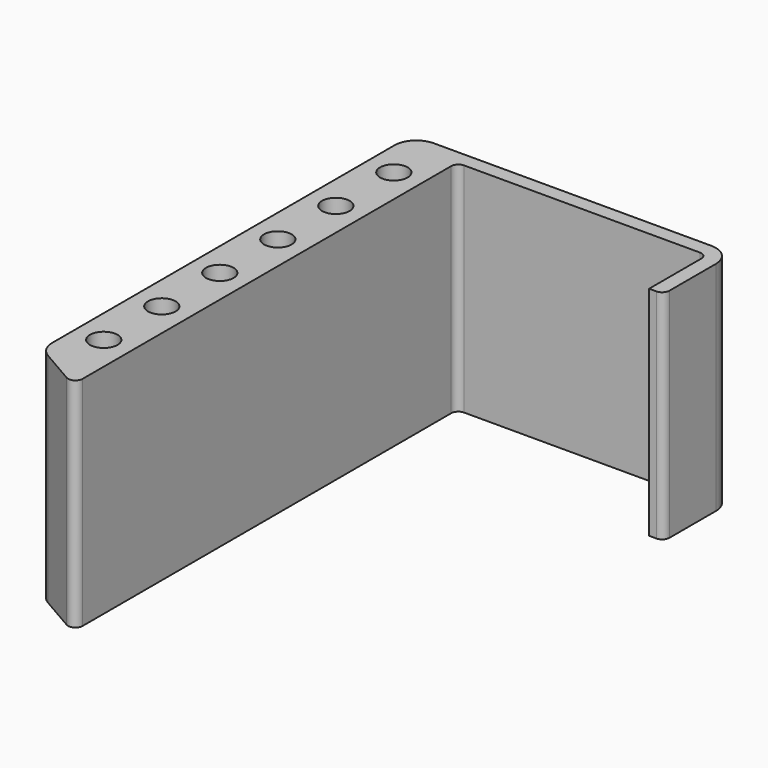
from build123d import *

# Parameters (mm, degrees)
F1_DEPTH  = 15
F2_R      = 1.9
F3_DEPTH  = 15
F4_R      = 1
F5_R      = 3
F7_R      = 1.9
F7_R_2    = 1.5
F8_DEPTH  = 1.6
F9_W      = 2
F9_H      = 58
F10_DEPTH = 12
F11_R     = 0.99999
F12_SIZE  = 0.39999


# Not quite as in the source:
# - a fillet or chamfer is up to 0.001 mm smaller than in the source, because OpenCascade refuses the exact size
# - a feature names something its author has since deleted; it is built from what else it names


with BuildPart() as f1:
    # F0 (on Top) → F1 (new body)
    with BuildSketch(Plane.XY):
        Polygon((-2, 2), (0, 0), (34.5, 0), (34.5, -10), (36.5, -10), (36.5, 2), align=None)
    extrude(amount=F1_DEPTH)

    # F2 (on Top) → F3 (join, through all)
    with BuildSketch(Plane.XY):
        Polygon((0, 0), (-2, 2), (-7.8, 2), (-7.8, -61.7483339502), (0, -66.2516660498), align=None)
        with Locations((-3.9, -56)):
            Circle(F2_R, mode=Mode.SUBTRACT)
        with Locations((-3.9, -46)):
            Circle(F2_R, mode=Mode.SUBTRACT)
        with Locations((-3.9, -36)):
            Circle(F2_R, mode=Mode.SUBTRACT)
        with Locations((-3.9, -26)):
            Circle(F2_R, mode=Mode.SUBTRACT)
        with Locations((-3.9, -16)):
            Circle(F2_R, mode=Mode.SUBTRACT)
        with Locations((-3.9, -6)):
            Circle(F2_R, mode=Mode.SUBTRACT)
    extrude(amount=F3_DEPTH)

    # F4
    f4_edges = [f1.edges().sort_by_distance(p)[0] for p in [
        (34.5, 0, 7.5),
        (0, -66.251666, 7.5),
        (36.5, -10, 7.5),
        (0, 0, 7.5),
    ]]
    fillet(f4_edges, radius=F4_R)

    # F5
    f5_edges = [f1.edges().sort_by_distance(p)[0] for p in [
        (36.5, 2, 7.5),
        (-7.8, 2, 7.5),
        (-7.8, -61.748334, 7.5),
    ]]
    fillet(f5_edges, radius=F5_R)

    # F7 (on offset) → F8 (join)
    with BuildSketch(Plane.XY.offset(4.8)):
        with Locations((-3.9, -6)):
            Circle(F7_R)
        with Locations((-3.9, -6)):
            Circle(F7_R_2, mode=Mode.SUBTRACT)
        with Locations((-3.9, -16)):
            Circle(F7_R)
        with Locations((-3.9, -16)):
            Circle(F7_R_2, mode=Mode.SUBTRACT)
        with Locations((-3.9, -26)):
            Circle(F7_R)
        with Locations((-3.9, -26)):
            Circle(F7_R_2, mode=Mode.SUBTRACT)
        with Locations((-3.9, -36)):
            Circle(F7_R)
        with Locations((-3.9, -36)):
            Circle(F7_R_2, mode=Mode.SUBTRACT)
        with Locations((-3.9, -46)):
            Circle(F7_R)
        with Locations((-3.9, -46)):
            Circle(F7_R_2, mode=Mode.SUBTRACT)
        with Locations((-3.9, -56)):
            Circle(F7_R)
        with Locations((-3.9, -56)):
            Circle(F7_R_2, mode=Mode.SUBTRACT)
    extrude(amount=-F8_DEPTH)

    # F9 (on face) → F10 (cut, through all)
    with BuildSketch(Plane(origin=(0, 0, 0), x_dir=(1, 0, 0), z_dir=(0, 0, -1))):
        with Locations((-3.9, 31)):
            Rectangle(F9_W, F9_H)
    extrude(amount=-F10_DEPTH, mode=Mode.SUBTRACT)

    # F11 (radius 1 in the source; OpenCascade refuses exactly that, so slightly less here)
    f11_edges = [f1.edges().sort_by_distance(p)[0] for p in [
        (-2.9, -2, 6),
        (-4.9, -2, 6),
        (-4.9, -3.192225, 12),
        (-2.9, -3.192225, 12),
        (-2.9, -11, 12),
        (-4.9, -11, 12),
        (-4.9, -21, 12),
        (-4.9, -31, 12),
        (-4.9, -41, 12),
        (-4.9, -51, 12),
        (-4.9, -58.807775, 12),
        (-4.9, -60, 6),
        (-3.9, -60, 12),
        (-2.9, -58.807775, 12),
        (-2.9, -60, 6),
        (-2.9, -51, 12),
        (-2.9, -41, 12),
        (-2.9, -31, 12),
        (-2.9, -21, 12),
        (-3.9, -2, 12),
    ]]
    fillet(f11_edges, radius=F11_R)

    # F12 (size 0.4 in the source; OpenCascade refuses exactly that, so slightly less here)
    f12_edges = [f1.edges().sort_by_distance(p)[0] for p in [
        (-2, -6, 3.2),
        (-2, -16, 3.2),
        (-2, -26, 3.2),
        (-2, -36, 3.2),
        (-2, -46, 3.2),
        (-2, -56, 3.2),
        (-5.8, -56, 3.2),
        (-5.8, -46, 3.2),
        (-5.8, -36, 3.2),
        (-5.8, -26, 3.2),
        (-5.8, -16, 3.2),
        (-5.8, -6, 3.2),
        (-5.8, -6, 4.8),
        (-5.8, -16, 4.8),
        (-5.8, -26, 4.8),
        (-5.8, -36, 4.8),
        (-5.8, -46, 4.8),
        (-5.8, -56, 4.8),
        (-2.240181, -5.075338, 4.8),
        (-2.240181, -6.924662, 4.8),
        (-2.240181, -15.075338, 4.8),
        (-2.240181, -16.924662, 4.8),
        (-2.240181, -25.075338, 4.8),
        (-2.240181, -26.924662, 4.8),
        (-2.240181, -35.075338, 4.8),
        (-2.240181, -36.924662, 4.8),
        (-2.240181, -45.075338, 4.8),
        (-2.240181, -46.924662, 4.8),
        (-2.240181, -55.075338, 4.8),
        (-2.240181, -56.924662, 4.8),
    ]]
    chamfer(f12_edges, length=F12_SIZE)

    # F13: F1 across face


with BuildPart() as f1_1:
    add(f1.part)
    add(f1.part.mirror(Plane(origin=(1.1887254371, -25.0161472082, 0), x_dir=(1, 0, 0), z_dir=(0, 0, -1))))


solid = f1_1.part
